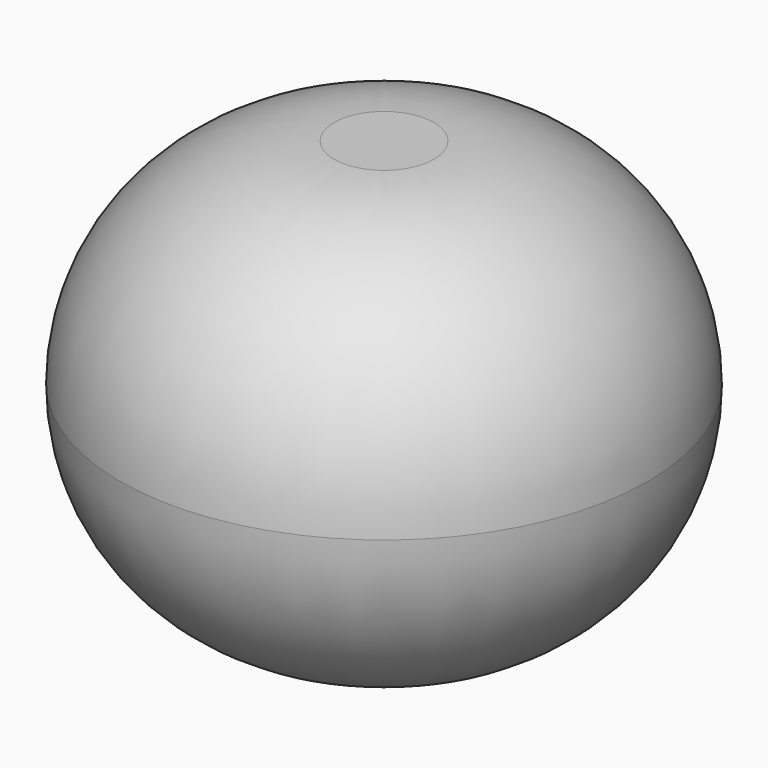
from build123d import *

# Parameters (mm, degrees)
F0_R     = 62.6417083558
F1_DEPTH = 101.6
F2_R     = 50.8
F3_R     = 50.79999


# Not quite as in the source:
# - a fillet or chamfer is up to 0.001 mm smaller than in the source, because OpenCascade refuses the exact size


with BuildPart() as f1:
    # F0 (on Top) → F1 (new body)
    with BuildSketch(Plane.XY):
        Circle(F0_R)
    extrude(amount=F1_DEPTH)

    # F2
    f2_edges = [f1.edges().sort_by_distance(p)[0] for p in [
        (-62.641708, 0, 101.6),
    ]]
    fillet(f2_edges, radius=F2_R)

    # F3 (radius 50.8 in the source; OpenCascade refuses exactly that, so slightly less here)
    f3_edges = [f1.edges().sort_by_distance(p)[0] for p in [
        (-62.641708, 0, 0),
    ]]
    fillet(f3_edges, radius=F3_R)


solid = f1.part
